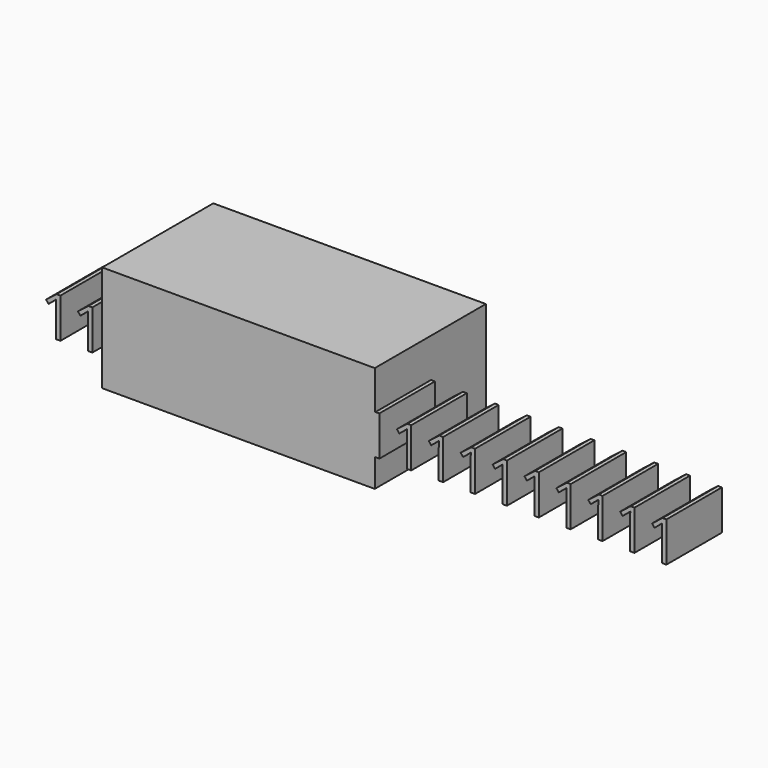
from build123d import *

# Parameters (mm, degrees)
F0_W         = 99.7177325189
F0_H         = 38.9101263136
F1_DEPTH     = 50.8
F2_TEXT_SIZE = 20.4094142343
F3_DEPTH     = 25.4


# Not quite as in the source:
# - Text() gives the source's letters only with a copy of the font that has no kerning and outlines rounded to 1/6400 em; it was checked with that copy


with BuildPart() as f1:
    # F0 (on Front) → F1 (new body)
    with BuildSketch(Plane.XZ):
        with Locations((-28.5509396344, 35.2868670598)):
            Rectangle(F0_W, F0_H)
    extrude(amount=F1_DEPTH)

    # F2 (on face) → F3 (join)
    with BuildSketch(Plane.XZ.offset(50.8)):
        with Locations((-100.8239239454, 26.1228028685)):
            Text('11111111111111111111', F2_TEXT_SIZE, font='Open Sans', text_align=(TextAlign.LEFT, TextAlign.BOTTOM))
    extrude(amount=-F3_DEPTH)


solid = f1.part
